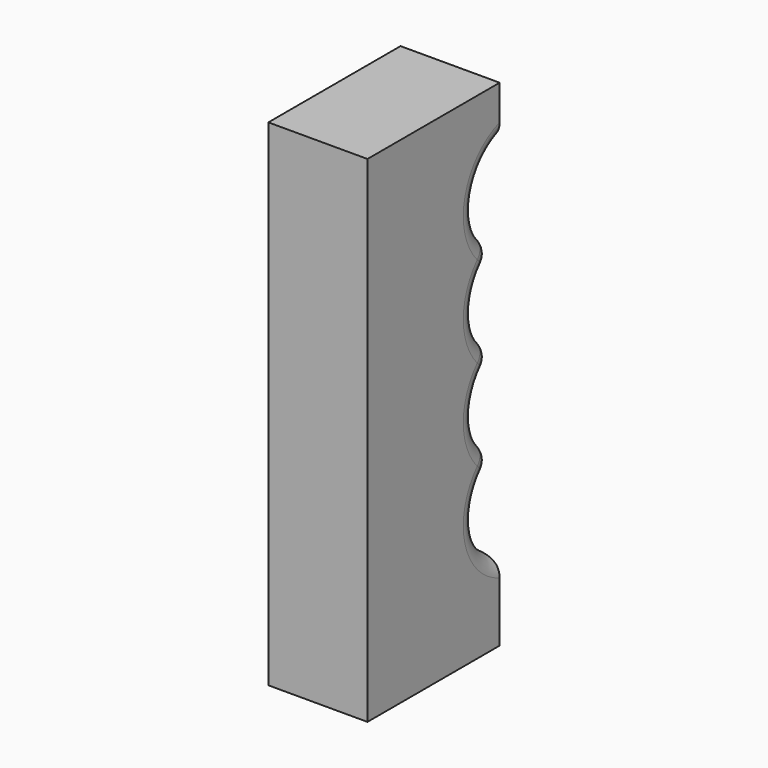
from build123d import *

# Parameters (mm, degrees)
F0_W     = 30.48
F0_H     = 152.4
F1_DEPTH = 50.8
F3_DEPTH = 30.481
F4_R     = 5.08


with BuildPart() as f1:
    # F0 (on Front) → F1 (new body)
    with BuildSketch(Plane.XZ):
        with Locations((0.2509840885, 76.2)):
            Rectangle(F0_W, F0_H)
    extrude(amount=-F1_DEPTH)

    # F2 (on face) → F3 (cut, through all)
    with BuildSketch(Plane.YZ.offset(15.4909840885)):
        with BuildLine():
            ThreePointArc((65.3252072253, 107.95), (71.4179823352, 113.7862789789), (73.66, 121.92))
            ThreePointArc((73.66, 121.92), (49.6512789789, 135.5529823352), (50.2447927747, 107.95))
            ThreePointArc((50.2447927747, 107.95), (57.785, 109.855), (65.3252072253, 107.95))
        make_face()
        with BuildLine():
            ThreePointArc((65.3252072253, 107.95), (57.785, 109.855), (50.2447927747, 107.95))
            ThreePointArc((50.2447927747, 107.95), (57.785, 106.045), (65.3252072253, 107.95))
        make_face()
        with BuildLine():
            ThreePointArc((65.3252072253, 107.95), (57.785, 106.045), (50.2447927747, 107.95))
            ThreePointArc((50.2447927747, 107.95), (41.91, 93.98), (50.2447927747, 80.01))
            ThreePointArc((50.2447927747, 80.01), (57.785, 81.915), (65.3252072253, 80.01))
            ThreePointArc((65.3252072253, 80.01), (71.4179823352, 85.8462789789), (73.66, 93.98))
            ThreePointArc((73.66, 93.98), (71.4179823352, 102.1137210211), (65.3252072253, 107.95))
        make_face()
        with BuildLine():
            ThreePointArc((65.3252072253, 80.01), (57.785, 81.915), (50.2447927747, 80.01))
            ThreePointArc((50.2447927747, 80.01), (57.785, 78.105), (65.3252072253, 80.01))
        make_face()
        with BuildLine():
            ThreePointArc((65.3252072253, 80.01), (57.785, 78.105), (50.2447927747, 80.01))
            ThreePointArc((50.2447927747, 80.01), (41.91, 66.04), (50.2447927747, 52.07))
            ThreePointArc((50.2447927747, 52.07), (57.785, 53.975), (65.3252072253, 52.07))
            ThreePointArc((65.3252072253, 52.07), (71.4179823352, 57.9062789789), (73.66, 66.04))
            ThreePointArc((73.66, 66.04), (71.4179823352, 74.1737210211), (65.3252072253, 80.01))
        make_face()
        with BuildLine():
            ThreePointArc((65.3252072253, 52.07), (57.785, 53.975), (50.2447927747, 52.07))
            ThreePointArc((50.2447927747, 52.07), (57.785, 50.165), (65.3252072253, 52.07))
        make_face()
        with BuildLine():
            ThreePointArc((65.3252072253, 52.07), (57.785, 50.165), (50.2447927747, 52.07))
            ThreePointArc((50.2447927747, 52.07), (49.6512789789, 24.4670176648), (73.66, 38.1))
            ThreePointArc((73.66, 38.1), (71.4179823352, 46.2337210211), (65.3252072253, 52.07))
        make_face()
    extrude(amount=-F3_DEPTH, mode=Mode.SUBTRACT)

    # F4
    f4_edges = [f1.edges().sort_by_distance(p)[0] for p in [
        (15.490984, 41.91307, 122.232205),
        (15.490984, 41.91307, 37.787795),
        (-14.989016, 41.91307, 122.232205),
        (-14.989016, 41.91, 93.98),
        (-14.989016, 41.91, 66.04),
        (-14.989016, 41.91307, 37.787795),
        (0.250984, 50.8, 23.844285),
        (0.250984, 50.8, 136.175715),
        (0.250984, 50.244793, 52.07),
        (15.490984, 41.91, 66.04),
        (0.250984, 50.244793, 80.01),
        (15.490984, 41.91, 93.98),
        (0.250984, 50.244793, 107.95),
    ]]
    fillet(f4_edges, radius=F4_R)


solid = f1.part
